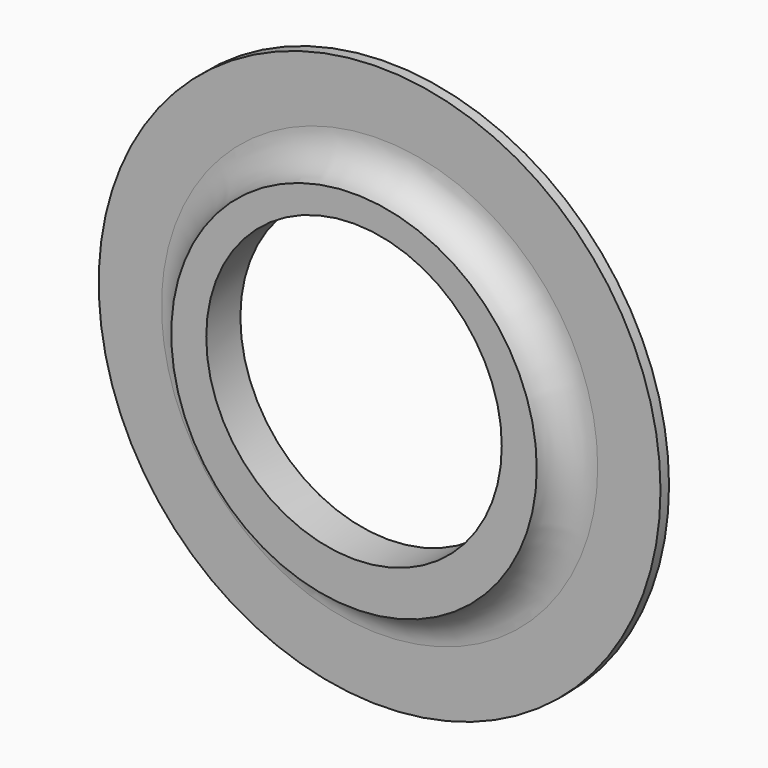
from build123d import *

# Parameters (mm, degrees)
F0_R     = 40.1475524572
F0_R_2   = 26.11755
F1_DEPTH = 1.524
F2_DEPTH = 6.096


# Not quite as in the source:
# - a fillet or chamfer that OpenCascade refuses, or shapes differently, is made with other operations: its cross-section is extruded or revolved along the edge and cut away or added


with BuildPart() as f1:
    # F0 (on Front) → F1 (new body)
    with BuildSketch(Plane.XZ):
        Circle(F0_R)
        with Locations((0.0001517863, 0)):
            Circle(F0_R_2, mode=Mode.SUBTRACT)
        with Locations((0.0001517863, 0)):
            Circle(F0_R_2)
        with BuildLine():
            ThreePointArc((0.0001517863, 22.3475835458), (14.93341969, 16.1620214495), (21.1189817863, 1.2287535458))
            ThreePointArc((21.1189817863, 1.2287535458), (-14.9331161175, -13.704514358), (0.0001517863, 22.3475835458))
        make_face(mode=Mode.SUBTRACT)
    extrude(amount=F1_DEPTH)

    # F0 (on Front) → F2 (join)
    with BuildSketch(Plane.XZ):
        with Locations((0.0001517863, 0)):
            Circle(F0_R_2)
        with BuildLine():
            ThreePointArc((0.0001517863, 22.3475835458), (14.93341969, 16.1620214495), (21.1189817863, 1.2287535458))
            ThreePointArc((21.1189817863, 1.2287535458), (-14.9331161175, -13.704514358), (0.0001517863, 22.3475835458))
        make_face(mode=Mode.SUBTRACT)
    extrude(amount=F2_DEPTH)

    # F3: fillet of radius 5.08 on 1 edges, made by hand

    # F3_s1 → F3_t2 (revolve)
    with BuildSketch(Plane.XY):
        with BuildLine():
            ThreePointArc((31.1722379668, -1.524), (27.764470369, -2.8365711686), (26.1177017863, -6.096))
            Line((26.1177017863, -6.096), (26.1177017863, -1.524))
            Line((26.1177017863, -1.524), (31.1722379668, -1.524))
        make_face()
    revolve(axis=Axis((0.0001517863, -1.524, 0), (0, 1, 0)))


solid = f1.part
